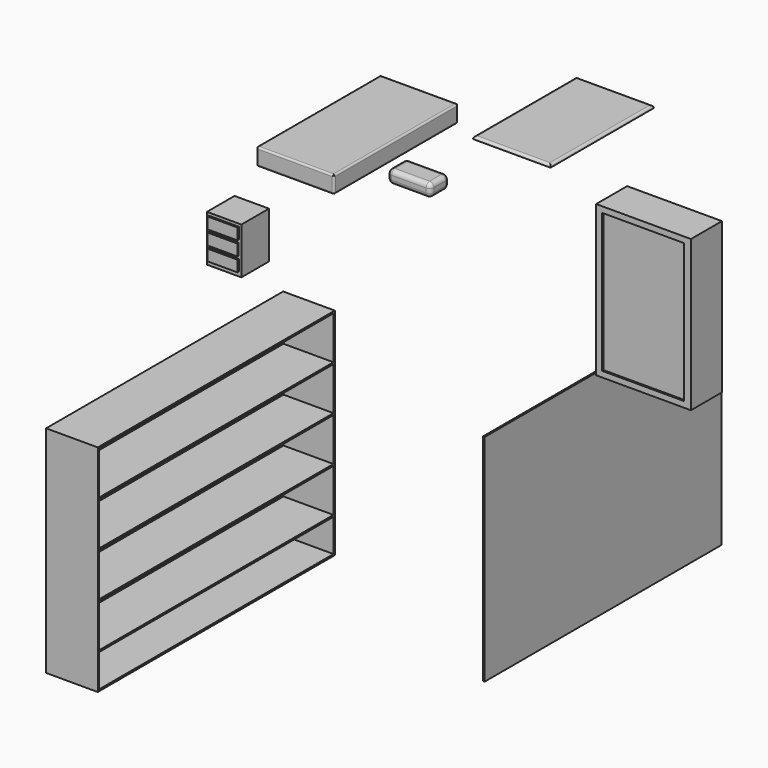
from build123d import *

# Parameters (mm, degrees)
F0_W         = 90
F0_H         = 180
F1_DEPTH     = 20
F2_R         = 2
F3_T1_DEPTH  = 21
F3_T3_DEPTH  = 86
F3_T5_DEPTH  = 176
F3_S9_W      = 2.04
F3_S9_H      = 2.04
F3_T10_DEPTH = 2.04
F3_S15_W     = 2.04
F3_S15_H     = 2.04
F3_T16_DEPTH = 2.04
F3_S21_W     = 2.04
F3_S21_H     = 2.04
F3_T22_DEPTH = 2.04
F3_S27_W     = 2.04
F3_S27_H     = 2.04
F3_T28_DEPTH = 2.04
F4_W         = 90
F4_H         = 150
F5_DEPTH     = 3
F6_R         = 2.99999
F7_W         = 50
F7_H         = 27
F8_DEPTH     = 15
F9_R         = 5
F10_W        = 110
F10_H        = 175
F11_DEPTH    = 45
F12_W        = 95.0341746211
F12_H        = 161.4808551967
F13_DEPTH    = 2
F14_W        = 344
F14_H        = 250
F15_DEPTH    = 60
F16_W        = 340
F16_H        = 50
F16_H_2      = 38
F17_DEPTH    = 58
F18_W        = 344
F18_H        = 250
F19_DEPTH    = 2
F20_W        = 40
F20_H        = 40
F21_DEPTH    = 54
F22_W        = 34.8343998194
F22_H        = 13.1596634164
F22_W_2      = 34.6408784389
F22_H_2      = 13.1596643478
F22_W_3      = 35.0279211998
F22_H_3      = 12.9661373794
F23_DEPTH    = 2


# Not quite as in the source:
# - a fillet or chamfer that OpenCascade refuses, or shapes differently, is made with other operations: its cross-section is extruded or revolved along the edge and cut away or added
# - a fillet or chamfer is up to 0.001 mm smaller than in the source, because OpenCascade refuses the exact size


with BuildPart() as f1:
    # F0 (on Top) → F1 (new body)
    with BuildSketch(Plane.XY):
        with Locations((-221.7077744007, 8.0266410112)):
            Rectangle(F0_W, F0_H)
    extrude(amount=F1_DEPTH)

    # F2
    f2_edges = [f1.edges().sort_by_distance(p)[0] for p in [
        (-221.707774, 98.026641, 20),
        (-266.707774, 8.026641, 20),
        (-221.707774, -81.973359, 20),
        (-176.707774, 8.026641, 20),
    ]]
    fillet(f2_edges, radius=F2_R)

    # F3: fillet of radius 2 on 16 edges, made by hand

    # F3_s2 → F3_t1 (cut)
    with BuildSketch(Plane.XY.offset(2)):
        with BuildLine():
            ThreePointArc((-266.7077744007, -79.9733589888), (-266.1219879631, -81.3875725511), (-264.7077744007, -81.9733589888))
            Line((-264.7077744007, -81.9733589888), (-266.7077744007, -81.9733589888))
            Line((-266.7077744007, -81.9733589888), (-266.7077744007, -79.9733589888))
        make_face()
        with BuildLine():
            ThreePointArc((-176.7077744007, -79.9733589888), (-177.2935608383, -81.3875725511), (-178.7077744007, -81.9733589888))
            Line((-178.7077744007, -81.9733589888), (-176.7077744007, -81.9733589888))
            Line((-176.7077744007, -81.9733589888), (-176.7077744007, -79.9733589888))
        make_face()
        with BuildLine():
            ThreePointArc((-178.7077744007, 98.0266410112), (-177.2935608383, 97.4408545736), (-176.7077744007, 96.0266410112))
            Line((-176.7077744007, 96.0266410112), (-176.7077744007, 98.0266410112))
            Line((-176.7077744007, 98.0266410112), (-178.7077744007, 98.0266410112))
        make_face()
        with BuildLine():
            ThreePointArc((-264.7077744007, 98.0266410112), (-266.1219879631, 97.4408545736), (-266.7077744007, 96.0266410112))
            Line((-266.7077744007, 96.0266410112), (-266.7077744007, 98.0266410112))
            Line((-266.7077744007, 98.0266410112), (-264.7077744007, 98.0266410112))
        make_face()
    extrude(amount=F3_T1_DEPTH, mode=Mode.SUBTRACT)

    # F3_s4 → F3_t3 (cut)
    with BuildSketch(Plane.YZ.offset(-264.7077744007)):
        with BuildLine():
            ThreePointArc((-79.9733589888, 0), (-81.3875725511, 0.5857864376), (-81.9733589888, 2))
            Line((-81.9733589888, 2), (-81.9733589888, 0))
            Line((-81.9733589888, 0), (-79.9733589888, 0))
        make_face()
        with BuildLine():
            ThreePointArc((98.0266410112, 2), (97.4408545736, 0.5857864376), (96.0266410112, 0))
            Line((96.0266410112, 0), (98.0266410112, 0))
            Line((98.0266410112, 0), (98.0266410112, 2))
        make_face()
    extrude(amount=F3_T3_DEPTH, mode=Mode.SUBTRACT)

    # F3_s6 → F3_t5 (cut)
    with BuildSketch(Plane.XZ.offset(-96.0266410112)):
        with BuildLine():
            ThreePointArc((-176.7077744007, 2), (-177.2935608383, 0.5857864376), (-178.7077744007, 0))
            Line((-178.7077744007, 0), (-176.7077744007, 0))
            Line((-176.7077744007, 0), (-176.7077744007, 2))
        make_face()
        with BuildLine():
            ThreePointArc((-264.7077744007, 0), (-266.1219879631, 0.5857864376), (-266.7077744007, 2))
            Line((-266.7077744007, 2), (-266.7077744007, 0))
            Line((-266.7077744007, 0), (-264.7077744007, 0))
        make_face()
    extrude(amount=F3_T5_DEPTH, mode=Mode.SUBTRACT)


with BuildPart() as f3_tool8:
    # F3_s9 → F3_t10 (new body)
    with BuildSketch(Plane.XY.offset(2)):
        with Locations((-265.7277744007, -80.9933589888)):
            Rectangle(F3_S9_W, F3_S9_H)
    extrude(amount=-F3_T10_DEPTH)

    # F3_s11 → F3_t12 (revolve, cut)
    with BuildSketch(Plane(origin=(-264.7077744007, -79.9733589888, 2), x_dir=(0.7071067812, 0.7071067812, 0), z_dir=(-0.7071067812, 0.7071067812, 0))):
        with BuildLine():
            ThreePointArc((0, -2), (2, 0), (0, 2))
            Line((0, 2), (0, -2))
        make_face()
    revolve(axis=Axis((-264.7077744007, -79.9733589888, 2), (0, 0, -1)), mode=Mode.SUBTRACT)


with BuildPart() as f1_1:
    add(f1.part)

    # F3_t7: cut F3_tool8
    add(f3_tool8.part, mode=Mode.SUBTRACT)


with BuildPart() as f3_tool14:
    # F3_s15 → F3_t16 (new body)
    with BuildSketch(Plane.YZ.offset(-178.7077744007)):
        with Locations((-80.9933589888, 0.98)):
            Rectangle(F3_S15_W, F3_S15_H)
    extrude(amount=F3_T16_DEPTH)

    # F3_s17 → F3_t18 (revolve, cut)
    with BuildSketch(Plane(origin=(-178.7077744007, -79.9733589888, 2), x_dir=(0, 0.7071067812, 0.7071067812), z_dir=(0, 0.7071067812, -0.7071067812))):
        with BuildLine():
            ThreePointArc((0, -2), (2, 0), (0, 2))
            Line((0, 2), (0, -2))
        make_face()
    revolve(axis=Axis((-178.7077744007, -79.9733589888, 2), (1, 0, 0)), mode=Mode.SUBTRACT)


with BuildPart() as f1_2:
    add(f1_1.part)

    # F3_t13: cut F3_tool14
    add(f3_tool14.part, mode=Mode.SUBTRACT)


with BuildPart() as f3_tool20:
    # F3_s21 → F3_t22 (new body)
    with BuildSketch(Plane.XZ.offset(-96.0266410112)):
        with Locations((-177.6877744007, 0.98)):
            Rectangle(F3_S21_W, F3_S21_H)
    extrude(amount=-F3_T22_DEPTH)

    # F3_s23 → F3_t24 (revolve, cut)
    with BuildSketch(Plane(origin=(-178.7077744007, 96.0266410112, 2), x_dir=(-0.7071067812, 0, 0.7071067812), z_dir=(-0.7071067812, 0, -0.7071067812))):
        with BuildLine():
            ThreePointArc((0, -2), (2, 0), (0, 2))
            Line((0, 2), (0, -2))
        make_face()
    revolve(axis=Axis((-178.7077744007, 96.0266410112, 2), (0, 1, 0)), mode=Mode.SUBTRACT)


with BuildPart() as f1_3:
    add(f1_2.part)

    # F3_t19: cut F3_tool20
    add(f3_tool20.part, mode=Mode.SUBTRACT)


with BuildPart() as f3_tool26:
    # F3_s27 → F3_t28 (new body)
    with BuildSketch(Plane.XZ.offset(-96.0266410112)):
        with Locations((-265.7277744007, 0.98)):
            Rectangle(F3_S27_W, F3_S27_H)
    extrude(amount=-F3_T28_DEPTH)

    # F3_s29 → F3_t30 (revolve, cut)
    with BuildSketch(Plane(origin=(-264.7077744007, 96.0266410112, 2), x_dir=(0.7071067812, 0, 0.7071067812), z_dir=(-0.7071067812, 0, 0.7071067812))):
        with BuildLine():
            ThreePointArc((0, -2), (2, 0), (0, 2))
            Line((0, 2), (0, -2))
        make_face()
    revolve(axis=Axis((-264.7077744007, 96.0266410112, 2), (0, 1, 0)), mode=Mode.SUBTRACT)


with BuildPart() as f1_4:
    add(f1_3.part)

    # F3_t25: cut F3_tool26
    add(f3_tool26.part, mode=Mode.SUBTRACT)


with BuildPart() as f5:
    # F4 (on Top) → F5 (new body)
    with BuildSketch(Plane.XY):
        with Locations((-101.6566661, 157.1905210614)):
            Rectangle(F4_W, F4_H)
    extrude(amount=F5_DEPTH)

    # F6 (radius 3 in the source; OpenCascade refuses exactly that, so slightly less here)
    f6_edges = [f5.edges().sort_by_distance(p)[0] for p in [
        (-101.656666, 82.190521, 3),
        (-56.656666, 157.190521, 3),
        (-101.656666, 232.190521, 3),
        (-146.656666, 157.190521, 3),
    ]]
    fillet(f6_edges, radius=F6_R)


with BuildPart() as f8:
    # F7 (on Top) → F8 (new body)
    with BuildSketch(Plane.XY):
        with Locations((-127.7489569783, -20.8424640596)):
            Rectangle(F7_W, F7_H)
    extrude(amount=F8_DEPTH)

    # F9
    f9_edges = [f8.edges().sort_by_distance(p)[0] for p in [
        (-127.748957, -7.342464, 15),
        (-152.748957, -20.842464, 15),
        (-127.748957, -34.342464, 15),
        (-102.748957, -20.842464, 15),
        (-152.748957, -34.342464, 7.5),
        (-102.748957, -34.342464, 7.5),
        (-127.748957, -34.342464, 0),
        (-127.748957, -7.342464, 0),
        (-152.748957, -20.842464, 0),
        (-102.748957, -20.842464, 0),
        (-152.748957, -7.342464, 7.5),
        (-102.748957, -7.342464, 7.5),
    ]]
    fillet(f9_edges, radius=F9_R)


with BuildPart() as f11:
    # F10 (on Front) → F11 (new body)
    with BuildSketch(Plane.XZ):
        with Locations((153.0910205841, -22.574326396)):
            Rectangle(F10_W, F10_H)
    extrude(amount=F11_DEPTH)

    # F12 (on face) → F13 (cut)
    with BuildSketch(Plane.XZ.offset(45)):
        with Locations((152.3183919489, -22.5743371993)):
            Rectangle(F12_W, F12_H)
    extrude(amount=-F13_DEPTH, mode=Mode.SUBTRACT)


with BuildPart() as f15:
    # F14 (on Right) → F15 (new body)
    with BuildSketch(Plane.YZ):
        with Locations((-548.5665888786, -46.5534925461)):
            Rectangle(F14_W, F14_H)
    extrude(amount=F15_DEPTH)

    # F16 (on face) → F17 (cut)
    with BuildSketch(Plane.YZ.offset(60)):
        with Locations((-548.5665888786, 51.4465074539)):
            Rectangle(F16_W, F16_H)
        with Locations((-548.5665888786, -0.5534925461)):
            Rectangle(F16_W, F16_H)
        with Locations((-548.5665888786, -52.5534925461)):
            Rectangle(F16_W, F16_H)
        with Locations((-548.5665888786, -104.5534925461)):
            Rectangle(F16_W, F16_H)
        with Locations((-548.5665888786, -150.5534925461)):
            Rectangle(F16_W, F16_H_2)
    extrude(amount=-F17_DEPTH, mode=Mode.SUBTRACT)


with BuildPart() as f19:
    # F18 (on Right) → F19 (new body)
    with BuildSketch(Plane.YZ):
        with Locations((85.2359144688, -312.5276565552)):
            Rectangle(F18_W, F18_H)
    extrude(amount=F19_DEPTH)


with BuildPart() as f21:
    # F20 (on Top) → F21 (new body)
    with BuildSketch(Plane.XY):
        with Locations((-225.745741725, -159.9699962139)):
            Rectangle(F20_W, F20_H)
    extrude(amount=-F21_DEPTH)

    # F22 (on face) → F23 (join)
    with BuildSketch(Plane.XZ.offset(179.9699962139)):
        with Locations((-226.0745540261, -9.7604426555)):
            Rectangle(F22_W, F22_H)
        with Locations((-226.1713147163, -26.2100240216)):
            Rectangle(F22_W_2, F22_H_2)
        with Locations((-226.1713147163, -42.5628405064)):
            Rectangle(F22_W_3, F22_H_3)
    extrude(amount=F23_DEPTH)


solid = Compound([f1_4.part, f5.part, f8.part, f11.part, f15.part, f19.part, f21.part])
